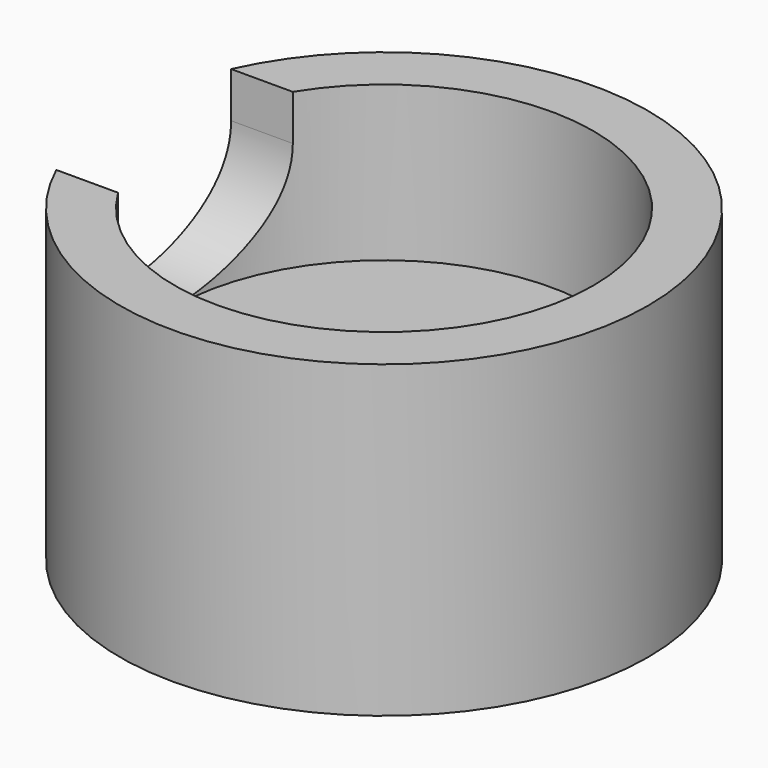
from build123d import *
from build123d import SkipClean  # not in build123d's __all__

# Parameters (mm, degrees)
F0_R     = 7.25
F1_DEPTH = 8.5
F2_R     = 5.75
F3_DEPTH = 4.25
F5_DEPTH = 25


with BuildPart() as f1:
    # F0 (on Top) → F1 (new body)
    with BuildSketch(Plane.XY):
        Circle(F0_R)
    extrude(amount=F1_DEPTH)

    # F2 (on face) → F3 (cut)
    with BuildSketch(Plane.XY.offset(8.5)):
        Circle(F2_R)
    extrude(amount=-F3_DEPTH, mode=Mode.SUBTRACT)

    # F4 (on Right) → F5 (cut)
    with BuildSketch(Plane.YZ):
        with BuildLine():
            Line((-3, 9.0031314455), (-3, 7.25))
            ThreePointArc((-3, 7.25), (0, 4.25), (3, 7.25))
            Line((3, 7.25), (3, 9.0439899638))
            Line((3, 9.0439899638), (-3, 9.0031314455))
        make_face()
    with SkipClean():  # cleaning this boolean's faces spoils the solid; the shape is the same uncleaned
        extrude(amount=-F5_DEPTH, mode=Mode.SUBTRACT)


solid = f1.part
